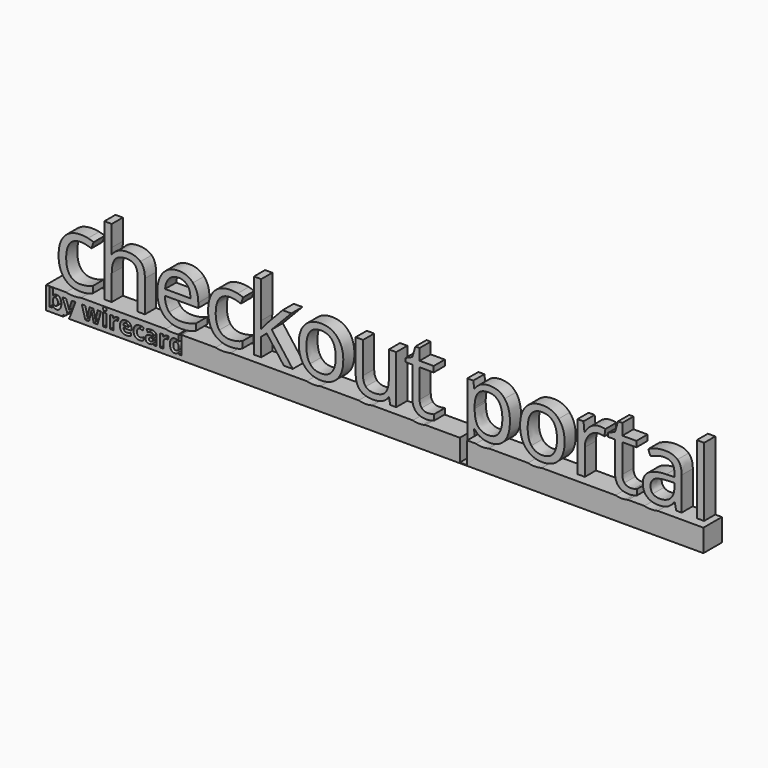
from build123d import *

# Parameters (mm, degrees)
F0_W         = 1.5870878906
F0_H         = 14.8709217956
F1_DEPTH     = 3
F2_DEPTH     = 5
F3_TEXT_SIZE = 4.9959736417
F4_DEPTH     = 2


# Not quite as in the source:
# - Text() gives the source's letters only with a copy of the font that has no kerning and outlines rounded to 1/6400 em; it was checked with that copy


with BuildPart() as f1:
    # F0 (on Front) → F1 (new body)
    with BuildSketch(Plane.XZ):
        with BuildLine():
            Line((-60.4767255251, 14.8709217956), (-60.4767255251, 0))
            Line((-60.4767255251, 0), (-58.8896376345, 0))
            Line((-58.8896376345, 0), (-58.8896376345, 5.4768293103))
            add(Edge.make_bspline(
                [(-58.1297313902, 8.4185991576), (-58.8896376345, 7.5195551502), (-58.8896376345, 5.4768293103)],
                knots=[0, 0, 0, 1, 1, 1], degree=2))
            add(Edge.make_bspline(
                [(-55.7185198261, 9.317643165), (-57.3698251458, 9.317643165), (-58.1297313902, 8.4185991576)],
                knots=[0, 0, 0, 1, 1, 1], degree=2))
            add(Edge.make_bspline(
                [(-53.8913810696, 8.6861717788), (-54.4739248908, 9.317643165), (-55.7185198261, 9.317643165)],
                knots=[0, 0, 0, 1, 1, 1], degree=2))
            add(Edge.make_bspline(
                [(-53.3088372485, 6.7764677563), (-53.3088372485, 8.0547003927), (-53.8913810696, 8.6861717788)],
                knots=[0, 0, 0, 1, 1, 1], degree=2))
            Line((-53.3088372485, 6.7764677563), (-53.3088372485, 0))
            Line((-53.3088372485, 0), (-51.721749358, 0))
            Line((-51.721749358, 0), (-51.721749358, 6.831511267))
            add(Edge.make_bspline(
                [(-52.683481808, 9.7319984813), (-51.721749358, 8.8191935962), (-51.721749358, 6.831511267)],
                knots=[0, 0, 0, 1, 1, 1], degree=2))
            add(Edge.make_bspline(
                [(-55.5656211854, 10.6448033663), (-53.6452142581, 10.6448033663), (-52.683481808, 9.7319984813)],
                knots=[0, 0, 0, 1, 1, 1], degree=2))
            add(Edge.make_bspline(
                [(-57.5380136506, 10.2105712267), (-56.6726073442, 10.6448033663), (-55.5656211854, 10.6448033663)],
                knots=[0, 0, 0, 1, 1, 1], degree=2))
            add(Edge.make_bspline(
                [(-58.8712897976, 9.021019802), (-58.403419957, 9.7763390871), (-57.5380136506, 10.2105712267)],
                knots=[0, 0, 0, 1, 1, 1], degree=2))
            Line((-58.8712897976, 9.021019802), (-58.9660869549, 9.021019802))
            add(Edge.make_bspline(
                [(-58.8896376345, 10.3695858131), (-58.8896376345, 9.5561650445), (-58.9660869549, 9.021019802)],
                knots=[0, 0, 0, 1, 1, 1], degree=2))
            Line((-58.8896376345, 10.3695858131), (-58.8896376345, 14.8709217956))
            Line((-58.8896376345, 14.8709217956), (-60.4767255251, 14.8709217956))
        make_face()
        with BuildLine():
            Line((-58.8896376345, 0), (-60.4767255251, 0))
            Line((-60.4767255251, 0), (-63.9066653381, 0))
            add(Edge.make_bspline(
                [(-63.9066653381, 0), (-64.6610084791, -0.1926522873), (-65.6080039074, -0.1926522873)],
                knots=[0.406741787, 0.406741787, 0.406741787, 1, 1, 1], degree=2))
            add(Edge.make_bspline(
                [(-65.6080039074, -0.1926522873), (-66.4518127873, -0.1926522873), (-67.1542872382, 0)],
                knots=[0, 0, 0, 0.3708835197, 0.3708835197, 0.3708835197], degree=2))
            Line((-67.1542872382, 0), (-71.4762537379, 0))
            Line((-71.4762537379, 0), (-71.4762537379, -4.8487260938))
            Line((-71.4762537379, -4.8487260938), (70.5573260784, -4.8487260938))
            Line((70.5573260784, -4.8487260938), (70.5573260784, 0))
            Line((70.5573260784, 0), (69.1171043692, 0))
            Line((69.1171043692, 0), (67.5300164786, 0))
            Line((67.5300164786, 0), (64.264101513, 0))
            Line((64.264101513, 0), (63.0867819795, 0))
            Line((63.0867819795, 0), (60.7063249973, 0))
            add(Edge.make_bspline(
                [(60.7063249973, 0), (60.0543585557, -0.1926522873), (59.1878666414, -0.1926522873)],
                knots=[0.2582329607, 0.2582329607, 0.2582329607, 1, 1, 1], degree=2))
            add(Edge.make_bspline(
                [(59.1878666414, -0.1926522873), (58.4260616691, -0.1926522873), (57.8254107013, 0)],
                knots=[0, 0, 0, 0.4894320446, 0.4894320446, 0.4894320446], degree=2))
            Line((57.8254107013, 0), (54.2992999583, 0))
            add(Edge.make_bspline(
                [(54.2992999583, 0), (54.0897603947, -0.0618327819), (53.7966605699, -0.1100870213)],
                knots=[0.4155624782, 0.4155624782, 0.4155624782, 1, 1, 1], degree=2))
            add(Edge.make_bspline(
                [(53.7966605699, -0.1100870213), (53.2951530284, -0.1926522873), (52.8915006169, -0.1926522873)],
                knots=[0, 0, 0, 1, 1, 1], degree=2))
            add(Edge.make_bspline(
                [(52.8915006169, -0.1926522873), (52.1466317843, -0.1926522873), (51.5844790179, 0)],
                knots=[0, 0, 0, 0.245299653, 0.245299653, 0.245299653], degree=2))
            Line((51.5844790179, 0), (43.3353355724, 0))
            Line((43.3353355724, 0), (41.7482476818, 0))
            Line((41.7482476818, 0), (35.6454867595, 0))
            add(Edge.make_bspline(
                [(35.6454867595, 0), (34.9450140523, -0.1926522873), (34.1124895647, -0.1926522873)],
                knots=[0.6340763655, 0.6340763655, 0.6340763655, 1, 1, 1], degree=2))
            add(Edge.make_bspline(
                [(34.1124895647, -0.1926522873), (33.3528022913, -0.1926522873), (32.6858735265, 0)],
                knots=[0, 0, 0, 0.5400617249, 0.5400617249, 0.5400617249], degree=2))
            Line((32.6858735265, 0), (24.1886250812, 0))
            add(Edge.make_bspline(
                [(24.1886250812, 0), (23.5581628048, -0.1926522873), (22.8071640705, -0.1926522873)],
                knots=[0.6329041565, 0.6329041565, 0.6329041565, 1, 1, 1], degree=2))
            add(Edge.make_bspline(
                [(22.8071640705, -0.1926522873), (22.0754941131, -0.1926522873), (21.4350805023, 0)],
                knots=[0, 0, 0, 0.714227875, 0.714227875, 0.714227875], degree=2))
            Line((21.4350805023, 0), (19.5134400115, 0))
            add(Edge.make_bspline(
                [(19.5134400115, 0), (19.5198432952, -0.1983221258), (19.5198432952, -0.3914205202)],
                knots=[0.7652569395, 0.7652569395, 0.7652569395, 1, 1, 1], degree=2))
            Line((19.5198432952, -0.3914205202), (19.5198432952, -4.7031621883))
            Line((19.5198432952, -4.7031621883), (17.9327554046, -4.7031621883))
            Line((17.9327554046, -4.7031621883), (17.9327554046, 0))
            Line((17.9327554046, 0), (10.4999553401, 0))
            add(Edge.make_bspline(
                [(10.4999553401, 0), (10.2904157764, -0.0618327819), (9.9973159517, -0.1100870213)],
                knots=[0.4155624782, 0.4155624782, 0.4155624782, 1, 1, 1], degree=2))
            add(Edge.make_bspline(
                [(9.9973159517, -0.1100870213), (9.4958084101, -0.1926522873), (9.0921559987, -0.1926522873)],
                knots=[0, 0, 0, 1, 1, 1], degree=2))
            add(Edge.make_bspline(
                [(9.0921559987, -0.1926522873), (8.3472871661, -0.1926522873), (7.7851343997, 0)],
                knots=[0, 0, 0, 0.245299653, 0.245299653, 0.245299653], degree=2))
            Line((7.7851343997, 0), (2.5756159315, 0))
            Line((2.5756159315, 0), (1.266803567, 0))
            Line((1.266803567, 0), (-0.9704054064, 0))
            add(Edge.make_bspline(
                [(-0.9704054064, 0), (-1.61552937, -0.1926522873), (-2.3752420547, -0.1926522873)],
                knots=[0.3156013684, 0.3156013684, 0.3156013684, 1, 1, 1], degree=2))
            add(Edge.make_bspline(
                [(-2.3752420547, -0.1926522873), (-3.2554913531, -0.1926522873), (-3.9317367984, 0)],
                knots=[0, 0, 0, 0.4605661865, 0.4605661865, 0.4605661865], degree=2))
            Line((-3.9317367984, 0), (-12.1750921094, 0))
            add(Edge.make_bspline(
                [(-12.1750921094, 0), (-12.8755648167, -0.1926522873), (-13.7080893043, -0.1926522873)],
                knots=[0.6340763655, 0.6340763655, 0.6340763655, 1, 1, 1], degree=2))
            add(Edge.make_bspline(
                [(-13.7080893043, -0.1926522873), (-14.4677765777, -0.1926522873), (-15.1347053424, 0)],
                knots=[0, 0, 0, 0.5400617249, 0.5400617249, 0.5400617249], degree=2))
            Line((-15.1347053424, 0), (-19.7842812861, 0))
            Line((-19.7842812861, 0), (-21.7046882135, 0))
            Line((-21.7046882135, 0), (-26.5974447162, 0))
            Line((-26.5974447162, 0), (-28.1661847699, 0))
            Line((-28.1661847699, 0), (-31.596124583, 0))
            add(Edge.make_bspline(
                [(-31.596124583, 0), (-32.3504677239, -0.1926522873), (-33.2974631522, -0.1926522873)],
                knots=[0.406741787, 0.406741787, 0.406741787, 1, 1, 1], degree=2))
            add(Edge.make_bspline(
                [(-33.2974631522, -0.1926522873), (-34.1412720322, -0.1926522873), (-34.843746483, 0)],
                knots=[0, 0, 0, 0.3708835197, 0.3708835197, 0.3708835197], degree=2))
            Line((-34.843746483, 0), (-42.0798203783, 0))
            add(Edge.make_bspline(
                [(-42.0798203783, 0), (-42.1552650705, -0.0178176726), (-42.2298017426, -0.033637701)],
                knots=[0.9005120931, 0.9005120931, 0.9005120931, 1, 1, 1], degree=2))
            add(Edge.make_bspline(
                [(-42.2298017426, -0.033637701), (-42.9790050821, -0.1926522873), (-44.0401216486, -0.1926522873)],
                knots=[0, 0, 0, 1, 1, 1], degree=2))
            add(Edge.make_bspline(
                [(-44.0401216486, -0.1926522873), (-44.896282125, -0.1926522873), (-45.6195000402, 0)],
                knots=[0, 0, 0, 0.3688754729, 0.3688754729, 0.3688754729], degree=2))
            Line((-45.6195000402, 0), (-51.721749358, 0))
            Line((-51.721749358, 0), (-53.3088372485, 0))
            Line((-53.3088372485, 0), (-58.8896376345, 0))
        make_face()
        with BuildLine():
            add(Edge.make_bspline(
                [(-63.9066653381, 0), (-64.6610084791, -0.1926522873), (-65.6080039074, -0.1926522873)],
                knots=[0.406741787, 0.406741787, 0.406741787, 1, 1, 1], degree=2))
            Line((-63.9066653381, 0), (-67.1542872382, 0))
            add(Edge.make_bspline(
                [(-65.6080039074, -0.1926522873), (-66.4518127873, -0.1926522873), (-67.1542872382, 0)],
                knots=[0, 0, 0, 0.3708835197, 0.3708835197, 0.3708835197], degree=2))
        make_face()
        with BuildLine():
            Line((-67.1542872382, 0), (-63.9066653381, 0))
            add(Edge.make_bspline(
                [(-62.9628574231, 0.3547248465), (-63.3894826503, 0.1320836929), (-63.9066653381, 0)],
                knots=[0, 0, 0, 0.406741787, 0.406741787, 0.406741787], degree=2))
            Line((-62.9628574231, 0.3547248465), (-62.9628574231, 1.7583343682))
            add(Edge.make_bspline(
                [(-65.647757554, 1.1956673704), (-64.3389451895, 1.1956673704), (-62.9628574231, 1.7583343682)],
                knots=[0, 0, 0, 1, 1, 1], degree=2))
            add(Edge.make_bspline(
                [(-67.9549980423, 2.2277331952), (-67.1767439611, 1.1956673704), (-65.647757554, 1.1956673704)],
                knots=[0, 0, 0, 1, 1, 1], degree=2))
            add(Edge.make_bspline(
                [(-68.7332521235, 5.1893798657), (-68.7332521235, 3.25979902), (-67.9549980423, 2.2277331952)],
                knots=[0, 0, 0, 1, 1, 1], degree=2))
            add(Edge.make_bspline(
                [(-65.5407285055, 9.2595416815), (-68.7332521235, 9.2595416815), (-68.7332521235, 5.1893798657)],
                knots=[0, 0, 0, 1, 1, 1], degree=2))
            add(Edge.make_bspline(
                [(-64.4429162651, 9.1219329048), (-65.0636847464, 9.2595416815), (-65.5407285055, 9.2595416815)],
                knots=[0, 0, 0, 1, 1, 1], degree=2))
            add(Edge.make_bspline(
                [(-63.2961764598, 8.773324004), (-63.8221477839, 8.9843241282), (-64.4429162651, 9.1219329048)],
                knots=[0, 0, 0, 1, 1, 1], degree=2))
            Line((-63.2961764598, 8.773324004), (-62.8099587824, 10.1188320423))
            add(Edge.make_bspline(
                [(-63.9933942615, 10.5026076305), (-63.2380749763, 10.3390060849), (-62.8099587824, 10.1188320423)],
                knots=[0, 0, 0, 1, 1, 1], degree=2))
            add(Edge.make_bspline(
                [(-65.5040328317, 10.666209176), (-64.7487135466, 10.666209176), (-63.9933942615, 10.5026076305)],
                knots=[0, 0, 0, 1, 1, 1], degree=2))
            add(Edge.make_bspline(
                [(-69.1109117661, 9.2320199262), (-67.8433820346, 10.666209176), (-65.5040328317, 10.666209176)],
                knots=[0, 0, 0, 1, 1, 1], degree=2))
            add(Edge.make_bspline(
                [(-70.3784414976, 5.1710320289), (-70.3784414976, 7.7978306763), (-69.1109117661, 9.2320199262)],
                knots=[0, 0, 0, 1, 1, 1], degree=2))
            add(Edge.make_bspline(
                [(-69.1307885894, 1.2078992616), (-70.3784414976, 2.6084508105), (-70.3784414976, 5.1710320289)],
                knots=[0, 0, 0, 1, 1, 1], degree=2))
            add(Edge.make_bspline(
                [(-67.1542872382, 0), (-68.3458695831, 0.3267892006), (-69.1307885894, 1.2078992616)],
                knots=[0.3708835197, 0.3708835197, 0.3708835197, 1, 1, 1], degree=2))
        make_face()
        with BuildLine():
            add(Edge.make_bspline(
                [(-45.6195000402, 0), (-46.8568839229, 0.3296168834), (-47.7051020665, 1.2231891257)],
                knots=[0.3688754729, 0.3688754729, 0.3688754729, 1, 1, 1], degree=2))
            Line((-45.6195000402, 0), (-42.0798203783, 0))
            add(Edge.make_bspline(
                [(-40.6396558792, 0.4862176775), (-41.3969347915, 0.1612761805), (-42.0798203783, 0)],
                knots=[0, 0, 0, 0.9005120931, 0.9005120931, 0.9005120931], degree=2))
            Line((-40.6396558792, 0.4862176775), (-40.6396558792, 1.9020590905))
            add(Edge.make_bspline(
                [(-43.9820201651, 1.1956673704), (-42.2909611989, 1.1956673704), (-40.6396558792, 1.9020590905)],
                knots=[0, 0, 0, 1, 1, 1], degree=2))
            add(Edge.make_bspline(
                [(-46.4712100359, 2.1512838748), (-45.5874558926, 1.1956673704), (-43.9820201651, 1.1956673704)],
                knots=[0, 0, 0, 1, 1, 1], degree=2))
            add(Edge.make_bspline(
                [(-47.4038917443, 4.9508579862), (-47.3549641792, 3.1069003793), (-46.4712100359, 2.1512838748)],
                knots=[0, 0, 0, 1, 1, 1], degree=2))
            Line((-47.4038917443, 4.9508579862), (-40.1901338755, 4.9508579862))
            Line((-40.1901338755, 4.9508579862), (-40.1901338755, 5.9538730693))
            add(Edge.make_bspline(
                [(-41.3368736808, 9.3711576892), (-40.1901338755, 8.0761062024), (-40.1901338755, 5.9538730693)],
                knots=[0, 0, 0, 1, 1, 1], degree=2))
            add(Edge.make_bspline(
                [(-44.4498900057, 10.666209176), (-42.4836134862, 10.666209176), (-41.3368736808, 9.3711576892)],
                knots=[0, 0, 0, 1, 1, 1], degree=2))
            add(Edge.make_bspline(
                [(-47.8014282101, 9.1754474291), (-46.5537753019, 10.666209176), (-44.4498900057, 10.666209176)],
                knots=[0, 0, 0, 1, 1, 1], degree=2))
            add(Edge.make_bspline(
                [(-49.0490811183, 5.1496262192), (-49.0490811183, 7.6846856822), (-47.8014282101, 9.1754474291)],
                knots=[0, 0, 0, 1, 1, 1], degree=2))
            add(Edge.make_bspline(
                [(-47.7051020665, 1.2231891257), (-49.0490811183, 2.6390305387), (-49.0490811183, 5.1496262192)],
                knots=[0, 0, 0, 1, 1, 1], degree=2))
        make_face()
        with BuildLine():
            add(Edge.make_bspline(
                [(-44.4712958154, 9.3359910018), (-45.7311806149, 9.3359910018), (-46.4819129408, 8.5149253012)],
                knots=[0, 0, 0, 1, 1, 1], degree=2))
            add(Edge.make_bspline(
                [(-42.5585338201, 8.5378600973), (-43.22670088, 9.3359910018), (-44.4712958154, 9.3359910018)],
                knots=[0, 0, 0, 1, 1, 1], degree=2))
            add(Edge.make_bspline(
                [(-41.8903667602, 6.2413225138), (-41.8903667602, 7.7397291928), (-42.5585338201, 8.5378600973)],
                knots=[0, 0, 0, 1, 1, 1], degree=2))
            Line((-41.8903667602, 6.2413225138), (-47.3671960705, 6.2413225138))
            add(Edge.make_bspline(
                [(-46.4819129408, 8.5149253012), (-47.2326452667, 7.6938596006), (-47.3671960705, 6.2413225138)],
                knots=[0, 0, 0, 1, 1, 1], degree=2))
        make_face(mode=Mode.SUBTRACT)
        with BuildLine():
            Line((-42.0798203783, 0), (-45.6195000402, 0))
            add(Edge.make_bspline(
                [(-44.0401216486, -0.1926522873), (-44.896282125, -0.1926522873), (-45.6195000402, 0)],
                knots=[0, 0, 0, 0.3688754729, 0.3688754729, 0.3688754729], degree=2))
            add(Edge.make_bspline(
                [(-42.2298017426, -0.033637701), (-42.9790050821, -0.1926522873), (-44.0401216486, -0.1926522873)],
                knots=[0, 0, 0, 1, 1, 1], degree=2))
            add(Edge.make_bspline(
                [(-42.0798203783, 0), (-42.1552650705, -0.0178176726), (-42.2298017426, -0.033637701)],
                knots=[0.9005120931, 0.9005120931, 0.9005120931, 1, 1, 1], degree=2))
        make_face()
        with BuildLine():
            add(Edge.make_bspline(
                [(-34.843746483, 0), (-36.0353288279, 0.3267892006), (-36.8202478342, 1.2078992616)],
                knots=[0.3708835197, 0.3708835197, 0.3708835197, 1, 1, 1], degree=2))
            Line((-34.843746483, 0), (-31.596124583, 0))
            add(Edge.make_bspline(
                [(-30.6523166679, 0.3547248465), (-31.0789418951, 0.1320836929), (-31.596124583, 0)],
                knots=[0, 0, 0, 0.406741787, 0.406741787, 0.406741787], degree=2))
            Line((-30.6523166679, 0.3547248465), (-30.6523166679, 1.7583343682))
            add(Edge.make_bspline(
                [(-33.3372167988, 1.1956673704), (-32.0284044343, 1.1956673704), (-30.6523166679, 1.7583343682)],
                knots=[0, 0, 0, 1, 1, 1], degree=2))
            add(Edge.make_bspline(
                [(-35.6444572871, 2.2277331952), (-34.8662032059, 1.1956673704), (-33.3372167988, 1.1956673704)],
                knots=[0, 0, 0, 1, 1, 1], degree=2))
            add(Edge.make_bspline(
                [(-36.4227113684, 5.1893798657), (-36.4227113684, 3.25979902), (-35.6444572871, 2.2277331952)],
                knots=[0, 0, 0, 1, 1, 1], degree=2))
            add(Edge.make_bspline(
                [(-33.2301877503, 9.2595416815), (-36.4227113684, 9.2595416815), (-36.4227113684, 5.1893798657)],
                knots=[0, 0, 0, 1, 1, 1], degree=2))
            add(Edge.make_bspline(
                [(-32.13237551, 9.1219329048), (-32.7531439913, 9.2595416815), (-33.2301877503, 9.2595416815)],
                knots=[0, 0, 0, 1, 1, 1], degree=2))
            add(Edge.make_bspline(
                [(-30.9856357047, 8.773324004), (-31.5116070287, 8.9843241282), (-32.13237551, 9.1219329048)],
                knots=[0, 0, 0, 1, 1, 1], degree=2))
            Line((-30.9856357047, 8.773324004), (-30.4994180272, 10.1188320423))
            add(Edge.make_bspline(
                [(-31.6828535063, 10.5026076305), (-30.9275342212, 10.3390060849), (-30.4994180272, 10.1188320423)],
                knots=[0, 0, 0, 1, 1, 1], degree=2))
            add(Edge.make_bspline(
                [(-33.1934920765, 10.666209176), (-32.4381727914, 10.666209176), (-31.6828535063, 10.5026076305)],
                knots=[0, 0, 0, 1, 1, 1], degree=2))
            add(Edge.make_bspline(
                [(-36.8003710109, 9.2320199262), (-35.5328412794, 10.666209176), (-33.1934920765, 10.666209176)],
                knots=[0, 0, 0, 1, 1, 1], degree=2))
            add(Edge.make_bspline(
                [(-38.0679007424, 5.1710320289), (-38.0679007424, 7.7978306763), (-36.8003710109, 9.2320199262)],
                knots=[0, 0, 0, 1, 1, 1], degree=2))
            add(Edge.make_bspline(
                [(-36.8202478342, 1.2078992616), (-38.0679007424, 2.6084508105), (-38.0679007424, 5.1710320289)],
                knots=[0, 0, 0, 1, 1, 1], degree=2))
        make_face()
        with BuildLine():
            Line((-31.596124583, 0), (-34.843746483, 0))
            add(Edge.make_bspline(
                [(-33.2974631522, -0.1926522873), (-34.1412720322, -0.1926522873), (-34.843746483, 0)],
                knots=[0, 0, 0, 0.3708835197, 0.3708835197, 0.3708835197], degree=2))
            add(Edge.make_bspline(
                [(-31.596124583, 0), (-32.3504677239, -0.1926522873), (-33.2974631522, -0.1926522873)],
                knots=[0.406741787, 0.406741787, 0.406741787, 1, 1, 1], degree=2))
        make_face()
        with Locations((68.3235604239, 7.4354608978)):
            Rectangle(F0_W, F0_H)
        with BuildLine():
            Line((-28.1661847699, 14.8709217956), (-28.1661847699, 0))
            Line((-28.1661847699, 0), (-26.5974447162, 0))
            Line((-26.5974447162, 0), (-26.5974447162, 3.917263175))
            Line((-26.5974447162, 3.917263175), (-25.4048353187, 4.9508579862))
            Line((-25.4048353187, 4.9508579862), (-21.7046882135, 0))
            Line((-21.7046882135, 0), (-19.7842812861, 0))
            Line((-19.7842812861, 0), (-24.3253709153, 6.0119745528))
            Line((-24.3253709153, 6.0119745528), (-20.0809046491, 10.4735568887))
            Line((-20.0809046491, 10.4735568887), (-21.9646159027, 10.4735568887))
            Line((-21.9646159027, 10.4735568887), (-25.3467338352, 6.8896127505))
            add(Edge.make_bspline(
                [(-26.5974447162, 5.3606263433), (-26.1876763591, 5.9446991509), (-25.3467338352, 6.8896127505)],
                knots=[0, 0, 0, 1, 1, 1], degree=2))
            Line((-26.5974447162, 5.3606263433), (-26.6738940366, 5.3606263433))
            add(Edge.make_bspline(
                [(-26.5974447162, 6.9844099077), (-26.5974447162, 6.4614965565), (-26.6738940366, 5.3606263433)],
                knots=[0, 0, 0, 1, 1, 1], degree=2))
            Line((-26.5974447162, 6.9844099077), (-26.5974447162, 14.8709217956))
            Line((-26.5974447162, 14.8709217956), (-28.1661847699, 14.8709217956))
        make_face()
        with BuildLine():
            Line((63.0867819795, 0), (64.264101513, 0))
            Line((64.264101513, 0), (64.264101513, 7.1495404397))
            add(Edge.make_bspline(
                [(63.3604705464, 9.8145637473), (64.264101513, 8.9843241282), (64.264101513, 7.1495404397)],
                knots=[0, 0, 0, 1, 1, 1], degree=2))
            add(Edge.make_bspline(
                [(60.5853602175, 10.6448033663), (62.4568395798, 10.6448033663), (63.3604705464, 9.8145637473)],
                knots=[0, 0, 0, 1, 1, 1], degree=2))
            add(Edge.make_bspline(
                [(58.7337576785, 10.4062814868), (59.655736482, 10.6448033663), (60.5853602175, 10.6448033663)],
                knots=[0, 0, 0, 1, 1, 1], degree=2))
            add(Edge.make_bspline(
                [(57.038111753, 9.7488173318), (57.811778875, 10.1677596073), (58.7337576785, 10.4062814868)],
                knots=[0, 0, 0, 1, 1, 1], degree=2))
            Line((57.038111753, 9.7488173318), (57.5273874032, 8.5348021245))
            add(Edge.make_bspline(
                [(60.4875050874, 9.3359910018), (59.1786927229, 9.3359910018), (57.5273874032, 8.5348021245)],
                knots=[0, 0, 0, 1, 1, 1], degree=2))
            add(Edge.make_bspline(
                [(62.1846799993, 8.7488602215), (61.6556507025, 9.3359910018), (60.4875050874, 9.3359910018)],
                knots=[0, 0, 0, 1, 1, 1], degree=2))
            add(Edge.make_bspline(
                [(62.7137092962, 6.929366397), (62.7137092962, 8.1617294412), (62.1846799993, 8.7488602215)],
                knots=[0, 0, 0, 1, 1, 1], degree=2))
            Line((62.7137092962, 6.929366397), (62.7137092962, 6.2780181876))
            Line((62.7137092962, 6.2780181876), (60.9370270911, 6.2199167041))
            add(Edge.make_bspline(
                [(55.8638501923, 2.8959002551), (55.8638501923, 6.0670180634), (60.9370270911, 6.2199167041)],
                knots=[0, 0, 0, 1, 1, 1], degree=2))
            add(Edge.make_bspline(
                [(56.7476043356, 0.6115945628), (55.8638501923, 1.415841413), (55.8638501923, 2.8959002551)],
                knots=[0, 0, 0, 1, 1, 1], degree=2))
            add(Edge.make_bspline(
                [(57.8254107013, 0), (57.1988208817, 0.2009718929), (56.7476043356, 0.6115945628)],
                knots=[0.4894320446, 0.4894320446, 0.4894320446, 1, 1, 1], degree=2))
            Line((57.8254107013, 0), (60.7063249973, 0))
            add(Edge.make_bspline(
                [(61.1342663376, 0.1574855999), (60.9332954821, 0.0670684567), (60.7063249973, 0)],
                knots=[0, 0, 0, 0.2582329607, 0.2582329607, 0.2582329607], degree=2))
            add(Edge.make_bspline(
                [(62.6953614593, 1.4922907333), (61.9125204189, 0.5076234872), (61.1342663376, 0.1574855999)],
                knots=[0, 0, 0, 1, 1, 1], degree=2))
            Line((62.6953614593, 1.4922907333), (62.7718107797, 1.4922907333))
            Line((62.7718107797, 1.4922907333), (63.0867819795, 0))
        make_face()
        with BuildLine():
            add(Edge.make_bspline(
                [(59.5028378412, 1.11921805), (60.9859546561, 1.11921805), (61.8314841393, 1.9311098322)],
                knots=[0, 0, 0, 1, 1, 1], degree=2))
            add(Edge.make_bspline(
                [(58.0472427817, 1.5672110673), (58.5670981601, 1.11921805), (59.5028378412, 1.11921805)],
                knots=[0, 0, 0, 1, 1, 1], degree=2))
            add(Edge.make_bspline(
                [(57.5273874032, 2.8775524182), (57.5273874032, 2.0152040846), (58.0472427817, 1.5672110673)],
                knots=[0, 0, 0, 1, 1, 1], degree=2))
            add(Edge.make_bspline(
                [(58.3622139815, 4.4967490233), (57.5273874032, 3.9753646585), (57.5273874032, 2.8775524182)],
                knots=[0, 0, 0, 1, 1, 1], degree=2))
            add(Edge.make_bspline(
                [(61.0899257318, 5.0854087901), (59.1970405598, 5.0181333882), (58.3622139815, 4.4967490233)],
                knots=[0, 0, 0, 1, 1, 1], degree=2))
            Line((61.0899257318, 5.0854087901), (62.6770136224, 5.1496262192))
            Line((62.6770136224, 5.1496262192), (62.6770136224, 4.2047126196))
            add(Edge.make_bspline(
                [(61.8314841393, 1.9311098322), (62.6770136224, 2.7430016144), (62.6770136224, 4.2047126196)],
                knots=[0, 0, 0, 1, 1, 1], degree=2))
        make_face(mode=Mode.SUBTRACT)
        with BuildLine():
            add(Edge.make_bspline(
                [(60.7063249973, 0), (60.0543585557, -0.1926522873), (59.1878666414, -0.1926522873)],
                knots=[0.2582329607, 0.2582329607, 0.2582329607, 1, 1, 1], degree=2))
            Line((60.7063249973, 0), (57.8254107013, 0))
            add(Edge.make_bspline(
                [(59.1878666414, -0.1926522873), (58.4260616691, -0.1926522873), (57.8254107013, 0)],
                knots=[0, 0, 0, 0.4894320446, 0.4894320446, 0.4894320446], degree=2))
        make_face()
        with BuildLine():
            add(Edge.make_bspline(
                [(-15.1347053424, 0), (-15.7026886887, 0.1640704324), (-16.2033951207, 0.4678698406)],
                knots=[0.5400617249, 0.5400617249, 0.5400617249, 1, 1, 1], degree=2))
            Line((-15.1347053424, 0), (-12.1750921094, 0))
            add(Edge.make_bspline(
                [(-10.1440219893, 1.2461239218), (-10.9613055526, 0.3338299323), (-12.1750921094, 0)],
                knots=[0, 0, 0, 0.6340763655, 0.6340763655, 0.6340763655], degree=2))
            add(Edge.make_bspline(
                [(-8.8550864481, 5.2474813492), (-8.8550864481, 2.6849001309), (-10.1440219893, 1.2461239218)],
                knots=[0, 0, 0, 1, 1, 1], degree=2))
            add(Edge.make_bspline(
                [(-10.1501379349, 9.2029691844), (-8.8550864481, 7.7397291928), (-8.8550864481, 5.2474813492)],
                knots=[0, 0, 0, 1, 1, 1], degree=2))
            add(Edge.make_bspline(
                [(-13.6408139023, 10.666209176), (-11.4451894217, 10.666209176), (-10.1501379349, 9.2029691844)],
                knots=[0, 0, 0, 1, 1, 1], degree=2))
            add(Edge.make_bspline(
                [(-17.1972362853, 9.2366068854), (-15.9159456761, 10.666209176), (-13.6408139023, 10.666209176)],
                knots=[0, 0, 0, 1, 1, 1], degree=2))
            add(Edge.make_bspline(
                [(-18.4785268944, 5.2474813492), (-18.4785268944, 7.8070045947), (-17.1972362853, 9.2366068854)],
                knots=[0, 0, 0, 1, 1, 1], degree=2))
            add(Edge.make_bspline(
                [(-17.8852801685, 2.3607550126), (-18.4785268944, 3.5931180567), (-18.4785268944, 5.2474813492)],
                knots=[0, 0, 0, 1, 1, 1], degree=2))
            add(Edge.make_bspline(
                [(-16.2033951207, 0.4678698406), (-17.2920334425, 1.1283919685), (-17.8852801685, 2.3607550126)],
                knots=[0, 0, 0, 1, 1, 1], degree=2))
        make_face()
        with BuildLine():
            add(Edge.make_bspline(
                [(-16.8333375204, 5.2474813492), (-16.8333375204, 3.2383932103), (-16.0306196567, 2.1879795486)],
                knots=[0, 0, 0, 1, 1, 1], degree=2))
            add(Edge.make_bspline(
                [(-16.0397935751, 8.2947512586), (-16.8333375204, 7.2718593522), (-16.8333375204, 5.2474813492)],
                knots=[0, 0, 0, 1, 1, 1], degree=2))
            add(Edge.make_bspline(
                [(-13.6897414674, 9.317643165), (-15.2462496298, 9.317643165), (-16.0397935751, 8.2947512586)],
                knots=[0, 0, 0, 1, 1, 1], degree=2))
            add(Edge.make_bspline(
                [(-11.3045226723, 8.2809903809), (-12.1118274952, 9.317643165), (-13.6897414674, 9.317643165)],
                knots=[0, 0, 0, 1, 1, 1], degree=2))
            add(Edge.make_bspline(
                [(-10.4972178493, 5.2474813492), (-10.4972178493, 7.2443375969), (-11.3045226723, 8.2809903809)],
                knots=[0, 0, 0, 1, 1, 1], degree=2))
            add(Edge.make_bspline(
                [(-11.3045226723, 2.1833925894), (-10.4972178493, 3.2292192918), (-10.4972178493, 5.2474813492)],
                knots=[0, 0, 0, 1, 1, 1], degree=2))
            add(Edge.make_bspline(
                [(-13.6713936305, 1.1375658869), (-12.1118274952, 1.1375658869), (-11.3045226723, 2.1833925894)],
                knots=[0, 0, 0, 1, 1, 1], degree=2))
            add(Edge.make_bspline(
                [(-16.0306196567, 2.1879795486), (-15.2279017929, 1.1375658869), (-13.6713936305, 1.1375658869)],
                knots=[0, 0, 0, 1, 1, 1], degree=2))
        make_face(mode=Mode.SUBTRACT)
        with BuildLine():
            Line((-12.1750921094, 0), (-15.1347053424, 0))
            add(Edge.make_bspline(
                [(-13.7080893043, -0.1926522873), (-14.4677765777, -0.1926522873), (-15.1347053424, 0)],
                knots=[0, 0, 0, 0.5400617249, 0.5400617249, 0.5400617249], degree=2))
            add(Edge.make_bspline(
                [(-12.1750921094, 0), (-12.8755648167, -0.1926522873), (-13.7080893043, -0.1926522873)],
                knots=[0.6340763655, 0.6340763655, 0.6340763655, 1, 1, 1], degree=2))
        make_face()
        with BuildLine():
            add(Edge.make_bspline(
                [(54.2992999583, 0), (54.0897603947, -0.0618327819), (53.7966605699, -0.1100870213)],
                knots=[0.4155624782, 0.4155624782, 0.4155624782, 1, 1, 1], degree=2))
            Line((54.2992999583, 0), (51.5844790179, 0))
            add(Edge.make_bspline(
                [(52.8915006169, -0.1926522873), (52.1466317843, -0.1926522873), (51.5844790179, 0)],
                knots=[0, 0, 0, 0.245299653, 0.245299653, 0.245299653], degree=2))
            add(Edge.make_bspline(
                [(53.7966605699, -0.1100870213), (53.2951530284, -0.1926522873), (52.8915006169, -0.1926522873)],
                knots=[0, 0, 0, 1, 1, 1], degree=2))
        make_face()
        with BuildLine():
            Line((51.5844790179, 0), (54.2992999583, 0))
            add(Edge.make_bspline(
                [(54.5550378278, 0.0947971572), (54.4482924119, 0.0439660068), (54.2992999583, 0)],
                knots=[0, 0, 0, 0.4155624782, 0.4155624782, 0.4155624782], degree=2))
            Line((54.5550378278, 0.0947971572), (54.5550378278, 1.3088123645))
            add(Edge.make_bspline(
                [(53.9342693465, 1.1803775063), (54.3256898668, 1.2415369626), (54.5550378278, 1.3088123645)],
                knots=[0, 0, 0, 1, 1, 1], degree=2))
            add(Edge.make_bspline(
                [(53.1208485779, 1.11921805), (53.5428488263, 1.11921805), (53.9342693465, 1.1803775063)],
                knots=[0, 0, 0, 1, 1, 1], degree=2))
            add(Edge.make_bspline(
                [(51.8884855338, 1.6253125508), (52.3380075375, 1.11921805), (53.1208485779, 1.11921805)],
                knots=[0, 0, 0, 1, 1, 1], degree=2))
            add(Edge.make_bspline(
                [(51.4389635301, 3.0763206511), (51.4389635301, 2.1314070515), (51.8884855338, 1.6253125508)],
                knots=[0, 0, 0, 1, 1, 1], degree=2))
            Line((51.4389635301, 3.0763206511), (51.4389635301, 9.2411938446))
            Line((51.4389635301, 9.2411938446), (54.4785885075, 9.2411938446))
            Line((54.4785885075, 9.2411938446), (54.4785885075, 10.4735568887))
            Line((54.4785885075, 10.4735568887), (51.4389635301, 10.4735568887))
            Line((51.4389635301, 10.4735568887), (51.4389635301, 12.9015873032))
            Line((51.4389635301, 12.9015873032), (50.5215716858, 12.9015873032))
            Line((50.5215716858, 12.9015873032), (49.8549336123, 10.666209176))
            Line((49.8549336123, 10.666209176), (48.3534689606, 10.0056870482))
            Line((48.3534689606, 10.0056870482), (48.3534689606, 9.2411938446))
            Line((48.3534689606, 9.2411938446), (49.8549336123, 9.2411938446))
            Line((49.8549336123, 9.2411938446), (49.8549336123, 3.0090452492))
            add(Edge.make_bspline(
                [(51.5844790179, 0), (49.8549336123, 0.5927230075), (49.8549336123, 3.0090452492)],
                knots=[0.245299653, 0.245299653, 0.245299653, 1, 1, 1], degree=2))
        make_face()
        with BuildLine():
            add(Edge.make_bspline(
                [(-3.9317367984, 0), (-4.723782915, 0.2256421793), (-5.2359756224, 0.7155656385)],
                knots=[0.4605661865, 0.4605661865, 0.4605661865, 1, 1, 1], degree=2))
            Line((-3.9317367984, 0), (-0.9704054064, 0))
            add(Edge.make_bspline(
                [(-0.3997916167, 0.2186450562), (-0.6729150312, 0.0888390518), (-0.9704054064, 0)],
                knots=[0, 0, 0, 0.3156013684, 0.3156013684, 0.3156013684], degree=2))
            add(Edge.make_bspline(
                [(0.9518323672, 1.4036095217), (0.4656146897, 0.6299423997), (-0.3997916167, 0.2186450562)],
                knots=[0, 0, 0, 1, 1, 1], degree=2))
            Line((0.9518323672, 1.4036095217), (1.037455606, 1.4036095217))
            Line((1.037455606, 1.4036095217), (1.266803567, 0))
            Line((1.266803567, 0), (2.5756159315, 0))
            Line((2.5756159315, 0), (2.5756159315, 10.4735568887))
            Line((2.5756159315, 10.4735568887), (0.9885280409, 10.4735568887))
            Line((0.9885280409, 10.4735568887), (0.9885280409, 4.9692058231))
            add(Edge.make_bspline(
                [(0.230150783, 2.0350809079), (0.9885280409, 2.9325959288), (0.9885280409, 4.9692058231)],
                knots=[0, 0, 0, 1, 1, 1], degree=2))
            add(Edge.make_bspline(
                [(-2.173415849, 1.1375658869), (-0.5282264749, 1.1375658869), (0.230150783, 2.0350809079)],
                knots=[0, 0, 0, 1, 1, 1], degree=2))
            add(Edge.make_bspline(
                [(-3.9974966327, 1.7675082866), (-3.4149528116, 1.1375658869), (-2.173415849, 1.1375658869)],
                knots=[0, 0, 0, 1, 1, 1], degree=2))
            add(Edge.make_bspline(
                [(-4.5800404538, 3.6787412955), (-4.5800404538, 2.3974506864), (-3.9974966327, 1.7675082866)],
                knots=[0, 0, 0, 1, 1, 1], degree=2))
            Line((-4.5800404538, 3.6787412955), (-4.5800404538, 10.4735568887))
            Line((-4.5800404538, 10.4735568887), (-6.1854761812, 10.4735568887))
            Line((-6.1854761812, 10.4735568887), (-6.1854761812, 3.620639812))
            add(Edge.make_bspline(
                [(-5.2359756224, 0.7155656385), (-6.1854761812, 1.6237835644), (-6.1854761812, 3.620639812)],
                knots=[0, 0, 0, 1, 1, 1], degree=2))
        make_face()
        with BuildLine():
            Line((-0.9704054064, 0), (-3.9317367984, 0))
            add(Edge.make_bspline(
                [(-2.3752420547, -0.1926522873), (-3.2554913531, -0.1926522873), (-3.9317367984, 0)],
                knots=[0, 0, 0, 0.4605661865, 0.4605661865, 0.4605661865], degree=2))
            add(Edge.make_bspline(
                [(-0.9704054064, 0), (-1.61552937, -0.1926522873), (-2.3752420547, -0.1926522873)],
                knots=[0.3156013684, 0.3156013684, 0.3156013684, 1, 1, 1], degree=2))
        make_face()
        with BuildLine():
            Line((41.7482476818, 0), (43.3353355724, 0))
            Line((43.3353355724, 0), (43.3353355724, 5.6205540326))
            add(Edge.make_bspline(
                [(44.2374375526, 8.1907801829), (43.3353355724, 7.1587143581), (43.3353355724, 5.6205540326)],
                knots=[0, 0, 0, 1, 1, 1], degree=2))
            add(Edge.make_bspline(
                [(46.4116562235, 9.2228460077), (45.1395395328, 9.2228460077), (44.2374375526, 8.1907801829)],
                knots=[0, 0, 0, 1, 1, 1], degree=2))
            add(Edge.make_bspline(
                [(47.5583960289, 9.0791212855), (46.9101057922, 9.2228460077), (46.4116562235, 9.2228460077)],
                knots=[0, 0, 0, 1, 1, 1], degree=2))
            Line((47.5583960289, 9.0791212855), (47.7785700715, 10.5500062091))
            add(Edge.make_bspline(
                [(46.5278591905, 10.666209176), (47.2250769921, 10.666209176), (47.7785700715, 10.5500062091)],
                knots=[0, 0, 0, 1, 1, 1], degree=2))
            add(Edge.make_bspline(
                [(44.7205972573, 10.1111871103), (45.5431919443, 10.666209176), (46.5278591905, 10.666209176)],
                knots=[0, 0, 0, 1, 1, 1], degree=2))
            add(Edge.make_bspline(
                [(43.3169877355, 8.5348021245), (43.8980025702, 9.5561650445), (44.7205972573, 10.1111871103)],
                knots=[0, 0, 0, 1, 1, 1], degree=2))
            Line((43.3169877355, 8.5348021245), (43.2405384152, 8.5348021245))
            Line((43.2405384152, 8.5348021245), (43.0570600463, 10.4735568887))
            Line((43.0570600463, 10.4735568887), (41.7482476818, 10.4735568887))
            Line((41.7482476818, 10.4735568887), (41.7482476818, 0))
        make_face()
        with BuildLine():
            add(Edge.make_bspline(
                [(35.6454867595, 0), (34.9450140523, -0.1926522873), (34.1124895647, -0.1926522873)],
                knots=[0.6340763655, 0.6340763655, 0.6340763655, 1, 1, 1], degree=2))
            Line((35.6454867595, 0), (32.6858735265, 0))
            add(Edge.make_bspline(
                [(34.1124895647, -0.1926522873), (33.3528022913, -0.1926522873), (32.6858735265, 0)],
                knots=[0, 0, 0, 0.5400617249, 0.5400617249, 0.5400617249], degree=2))
        make_face()
        with BuildLine():
            Line((32.6858735265, 0), (35.6454867595, 0))
            add(Edge.make_bspline(
                [(37.6765568797, 1.2461239218), (36.8592733163, 0.3338299323), (35.6454867595, 0)],
                knots=[0, 0, 0, 0.6340763655, 0.6340763655, 0.6340763655], degree=2))
            add(Edge.make_bspline(
                [(38.9654924209, 5.2474813492), (38.9654924209, 2.6849001309), (37.6765568797, 1.2461239218)],
                knots=[0, 0, 0, 1, 1, 1], degree=2))
            add(Edge.make_bspline(
                [(37.670440934, 9.2029691844), (38.9654924209, 7.7397291928), (38.9654924209, 5.2474813492)],
                knots=[0, 0, 0, 1, 1, 1], degree=2))
            add(Edge.make_bspline(
                [(34.1797649666, 10.666209176), (36.3753894472, 10.666209176), (37.670440934, 9.2029691844)],
                knots=[0, 0, 0, 1, 1, 1], degree=2))
            add(Edge.make_bspline(
                [(30.6233425836, 9.2366068854), (31.9046331928, 10.666209176), (34.1797649666, 10.666209176)],
                knots=[0, 0, 0, 1, 1, 1], degree=2))
            add(Edge.make_bspline(
                [(29.3420519745, 5.2474813492), (29.3420519745, 7.8070045947), (30.6233425836, 9.2366068854)],
                knots=[0, 0, 0, 1, 1, 1], degree=2))
            add(Edge.make_bspline(
                [(29.9352987004, 2.3607550126), (29.3420519745, 3.5931180567), (29.3420519745, 5.2474813492)],
                knots=[0, 0, 0, 1, 1, 1], degree=2))
            add(Edge.make_bspline(
                [(31.6171837483, 0.4678698406), (30.5285454264, 1.1283919685), (29.9352987004, 2.3607550126)],
                knots=[0, 0, 0, 1, 1, 1], degree=2))
            add(Edge.make_bspline(
                [(32.6858735265, 0), (32.1178901803, 0.1640704324), (31.6171837483, 0.4678698406)],
                knots=[0.5400617249, 0.5400617249, 0.5400617249, 1, 1, 1], degree=2))
        make_face()
        with BuildLine():
            add(Edge.make_bspline(
                [(30.9872413485, 5.2474813492), (30.9872413485, 3.2383932103), (31.7899592123, 2.1879795486)],
                knots=[0, 0, 0, 1, 1, 1], degree=2))
            add(Edge.make_bspline(
                [(31.7807852938, 8.2947512586), (30.9872413485, 7.2718593522), (30.9872413485, 5.2474813492)],
                knots=[0, 0, 0, 1, 1, 1], degree=2))
            add(Edge.make_bspline(
                [(34.1308374016, 9.317643165), (32.5743292391, 9.317643165), (31.7807852938, 8.2947512586)],
                knots=[0, 0, 0, 1, 1, 1], degree=2))
            add(Edge.make_bspline(
                [(36.5160561967, 8.2809903809), (35.7087513737, 9.317643165), (34.1308374016, 9.317643165)],
                knots=[0, 0, 0, 1, 1, 1], degree=2))
            add(Edge.make_bspline(
                [(37.3233610196, 5.2474813492), (37.3233610196, 7.2443375969), (36.5160561967, 8.2809903809)],
                knots=[0, 0, 0, 1, 1, 1], degree=2))
            add(Edge.make_bspline(
                [(36.5160561967, 2.1833925894), (37.3233610196, 3.2292192918), (37.3233610196, 5.2474813492)],
                knots=[0, 0, 0, 1, 1, 1], degree=2))
            add(Edge.make_bspline(
                [(34.1491852385, 1.1375658869), (35.7087513737, 1.1375658869), (36.5160561967, 2.1833925894)],
                knots=[0, 0, 0, 1, 1, 1], degree=2))
            add(Edge.make_bspline(
                [(31.7899592123, 2.1879795486), (32.592677076, 1.1375658869), (34.1491852385, 1.1375658869)],
                knots=[0, 0, 0, 1, 1, 1], degree=2))
        make_face(mode=Mode.SUBTRACT)
        with BuildLine():
            add(Edge.make_bspline(
                [(7.7851343997, 0), (6.0555889941, 0.5927230075), (6.0555889941, 3.0090452492)],
                knots=[0.245299653, 0.245299653, 0.245299653, 1, 1, 1], degree=2))
            Line((7.7851343997, 0), (10.4999553401, 0))
            add(Edge.make_bspline(
                [(10.7556932096, 0.0947971572), (10.6489477937, 0.0439660068), (10.4999553401, 0)],
                knots=[0, 0, 0, 0.4155624782, 0.4155624782, 0.4155624782], degree=2))
            Line((10.7556932096, 0.0947971572), (10.7556932096, 1.3088123645))
            add(Edge.make_bspline(
                [(10.1349247283, 1.1803775063), (10.5263452485, 1.2415369626), (10.7556932096, 1.3088123645)],
                knots=[0, 0, 0, 1, 1, 1], degree=2))
            add(Edge.make_bspline(
                [(9.3215039597, 1.11921805), (9.7435042081, 1.11921805), (10.1349247283, 1.1803775063)],
                knots=[0, 0, 0, 1, 1, 1], degree=2))
            add(Edge.make_bspline(
                [(8.0891409156, 1.6253125508), (8.5386629193, 1.11921805), (9.3215039597, 1.11921805)],
                knots=[0, 0, 0, 1, 1, 1], degree=2))
            add(Edge.make_bspline(
                [(7.6396189119, 3.0763206511), (7.6396189119, 2.1314070515), (8.0891409156, 1.6253125508)],
                knots=[0, 0, 0, 1, 1, 1], degree=2))
            Line((7.6396189119, 3.0763206511), (7.6396189119, 9.2411938446))
            Line((7.6396189119, 9.2411938446), (10.6792438892, 9.2411938446))
            Line((10.6792438892, 9.2411938446), (10.6792438892, 10.4735568887))
            Line((10.6792438892, 10.4735568887), (7.6396189119, 10.4735568887))
            Line((7.6396189119, 10.4735568887), (7.6396189119, 12.9015873032))
            Line((7.6396189119, 12.9015873032), (6.7222270676, 12.9015873032))
            Line((6.7222270676, 12.9015873032), (6.0555889941, 10.666209176))
            Line((6.0555889941, 10.666209176), (4.5541243423, 10.0056870482))
            Line((4.5541243423, 10.0056870482), (4.5541243423, 9.2411938446))
            Line((4.5541243423, 9.2411938446), (6.0555889941, 9.2411938446))
            Line((6.0555889941, 9.2411938446), (6.0555889941, 3.0090452492))
        make_face()
        with BuildLine():
            Line((10.4999553401, 0), (7.7851343997, 0))
            add(Edge.make_bspline(
                [(9.0921559987, -0.1926522873), (8.3472871661, -0.1926522873), (7.7851343997, 0)],
                knots=[0, 0, 0, 0.245299653, 0.245299653, 0.245299653], degree=2))
            add(Edge.make_bspline(
                [(9.9973159517, -0.1100870213), (9.4958084101, -0.1926522873), (9.0921559987, -0.1926522873)],
                knots=[0, 0, 0, 1, 1, 1], degree=2))
            add(Edge.make_bspline(
                [(10.4999553401, 0), (10.2904157764, -0.0618327819), (9.9973159517, -0.1100870213)],
                knots=[0.4155624782, 0.4155624782, 0.4155624782, 1, 1, 1], degree=2))
        make_face()
        with BuildLine():
            add(Edge.make_bspline(
                [(24.1886250812, 0), (23.5581628048, -0.1926522873), (22.8071640705, -0.1926522873)],
                knots=[0.6329041565, 0.6329041565, 0.6329041565, 1, 1, 1], degree=2))
            Line((24.1886250812, 0), (21.4350805023, 0))
            add(Edge.make_bspline(
                [(22.8071640705, -0.1926522873), (22.0754941131, -0.1926522873), (21.4350805023, 0)],
                knots=[0, 0, 0, 0.714227875, 0.714227875, 0.714227875], degree=2))
        make_face()
        with BuildLine():
            Line((21.4350805023, 0), (24.1886250812, 0))
            add(Edge.make_bspline(
                [(26.0042746478, 1.2369500034), (25.2755951529, 0.3321487714), (24.1886250812, 0)],
                knots=[0, 0, 0, 0.6329041565, 0.6329041565, 0.6329041565], degree=2))
            add(Edge.make_bspline(
                [(27.1556014123, 5.2474813492), (27.1556014123, 2.666552294), (26.0042746478, 1.2369500034)],
                knots=[0, 0, 0, 1, 1, 1], degree=2))
            add(Edge.make_bspline(
                [(26.0226224846, 9.2411938446), (27.1556014123, 7.8161785132), (27.1556014123, 5.2474813492)],
                knots=[0, 0, 0, 1, 1, 1], degree=2))
            add(Edge.make_bspline(
                [(22.8071640705, 10.666209176), (24.889643557, 10.666209176), (26.0226224846, 9.2411938446)],
                knots=[0, 0, 0, 1, 1, 1], degree=2))
            add(Edge.make_bspline(
                [(20.9433296402, 10.2839625743), (21.7552214224, 10.666209176), (22.8071640705, 10.666209176)],
                knots=[0, 0, 0, 1, 1, 1], degree=2))
            add(Edge.make_bspline(
                [(19.5198432952, 9.0393676389), (20.131437858, 9.9017159725), (20.9433296402, 10.2839625743)],
                knots=[0, 0, 0, 1, 1, 1], degree=2))
            Line((19.5198432952, 9.0393676389), (19.4433939748, 9.0393676389))
            Line((19.4433939748, 9.0393676389), (19.2232199322, 10.4735568887))
            Line((19.2232199322, 10.4735568887), (17.9327554046, 10.4735568887))
            Line((17.9327554046, 10.4735568887), (17.9327554046, 0))
            Line((17.9327554046, 0), (19.5134400115, 0))
            add(Edge.make_bspline(
                [(19.4036403282, 1.3485660111), (19.4925654551, 0.646525536), (19.5134400115, 0)],
                knots=[0, 0, 0, 0.7652569395, 0.7652569395, 0.7652569395], degree=2))
            Line((19.4036403282, 1.3485660111), (19.5198432952, 1.3485660111))
            add(Edge.make_bspline(
                [(20.9372136946, 0.1850073553), (20.0916842114, 0.5626669978), (19.5198432952, 1.3485660111)],
                knots=[0, 0, 0, 1, 1, 1], degree=2))
            add(Edge.make_bspline(
                [(21.4350805023, 0), (21.1788424517, 0.0770827567), (20.9372136946, 0.1850073553)],
                knots=[0.714227875, 0.714227875, 0.714227875, 1, 1, 1], degree=2))
        make_face()
        with BuildLine():
            add(Edge.make_bspline(
                [(22.5778161094, 9.317643165), (20.9723803819, 9.317643165), (20.255285757, 8.4293020624)],
                knots=[0, 0, 0, 1, 1, 1], degree=2))
            add(Edge.make_bspline(
                [(24.7413318755, 8.2718164625), (23.9722517127, 9.317643165), (22.5778161094, 9.317643165)],
                knots=[0, 0, 0, 1, 1, 1], degree=2))
            add(Edge.make_bspline(
                [(25.5104120383, 5.2658291861), (25.5104120383, 7.22598976), (24.7413318755, 8.2718164625)],
                knots=[0, 0, 0, 1, 1, 1], degree=2))
            add(Edge.make_bspline(
                [(24.7413318755, 2.2369071136), (25.5104120383, 3.3362483403), (25.5104120383, 5.2658291861)],
                knots=[0, 0, 0, 1, 1, 1], degree=2))
            add(Edge.make_bspline(
                [(22.6145117832, 1.1375658869), (23.9722517127, 1.1375658869), (24.7413318755, 2.2369071136)],
                knots=[0, 0, 0, 1, 1, 1], degree=2))
            add(Edge.make_bspline(
                [(20.255285757, 2.0885954321), (20.9907282188, 1.1375658869), (22.6145117832, 1.1375658869)],
                knots=[0, 0, 0, 1, 1, 1], degree=2))
            add(Edge.make_bspline(
                [(19.5198432952, 5.2474813492), (19.5198432952, 3.0396249773), (20.255285757, 2.0885954321)],
                knots=[0, 0, 0, 1, 1, 1], degree=2))
            Line((19.5198432952, 5.2474813492), (19.5198432952, 5.5991482229))
            add(Edge.make_bspline(
                [(20.255285757, 8.4293020624), (19.5381911321, 7.5409609599), (19.5198432952, 5.5991482229)],
                knots=[0, 0, 0, 1, 1, 1], degree=2))
        make_face(mode=Mode.SUBTRACT)
        with BuildLine():
            Line((19.5134400115, 0), (17.9327554046, 0))
            Line((17.9327554046, 0), (17.9327554046, -4.7031621883))
            Line((17.9327554046, -4.7031621883), (19.5198432952, -4.7031621883))
            Line((19.5198432952, -4.7031621883), (19.5198432952, -0.3914205202))
            add(Edge.make_bspline(
                [(19.5134400115, 0), (19.5198432952, -0.1983221258), (19.5198432952, -0.3914205202)],
                knots=[0.7652569395, 0.7652569395, 0.7652569395, 1, 1, 1], degree=2))
        make_face()
    extrude(amount=F1_DEPTH)

    # F0 (on Front) → F2 (join)
    with BuildSketch(Plane.XZ):
        with BuildLine():
            Line((-58.8896376345, 0), (-60.4767255251, 0))
            Line((-60.4767255251, 0), (-63.9066653381, 0))
            add(Edge.make_bspline(
                [(-63.9066653381, 0), (-64.6610084791, -0.1926522873), (-65.6080039074, -0.1926522873)],
                knots=[0.406741787, 0.406741787, 0.406741787, 1, 1, 1], degree=2))
            add(Edge.make_bspline(
                [(-65.6080039074, -0.1926522873), (-66.4518127873, -0.1926522873), (-67.1542872382, 0)],
                knots=[0, 0, 0, 0.3708835197, 0.3708835197, 0.3708835197], degree=2))
            Line((-67.1542872382, 0), (-71.4762537379, 0))
            Line((-71.4762537379, 0), (-71.4762537379, -4.8487260938))
            Line((-71.4762537379, -4.8487260938), (70.5573260784, -4.8487260938))
            Line((70.5573260784, -4.8487260938), (70.5573260784, 0))
            Line((70.5573260784, 0), (69.1171043692, 0))
            Line((69.1171043692, 0), (67.5300164786, 0))
            Line((67.5300164786, 0), (64.264101513, 0))
            Line((64.264101513, 0), (63.0867819795, 0))
            Line((63.0867819795, 0), (60.7063249973, 0))
            add(Edge.make_bspline(
                [(60.7063249973, 0), (60.0543585557, -0.1926522873), (59.1878666414, -0.1926522873)],
                knots=[0.2582329607, 0.2582329607, 0.2582329607, 1, 1, 1], degree=2))
            add(Edge.make_bspline(
                [(59.1878666414, -0.1926522873), (58.4260616691, -0.1926522873), (57.8254107013, 0)],
                knots=[0, 0, 0, 0.4894320446, 0.4894320446, 0.4894320446], degree=2))
            Line((57.8254107013, 0), (54.2992999583, 0))
            add(Edge.make_bspline(
                [(54.2992999583, 0), (54.0897603947, -0.0618327819), (53.7966605699, -0.1100870213)],
                knots=[0.4155624782, 0.4155624782, 0.4155624782, 1, 1, 1], degree=2))
            add(Edge.make_bspline(
                [(53.7966605699, -0.1100870213), (53.2951530284, -0.1926522873), (52.8915006169, -0.1926522873)],
                knots=[0, 0, 0, 1, 1, 1], degree=2))
            add(Edge.make_bspline(
                [(52.8915006169, -0.1926522873), (52.1466317843, -0.1926522873), (51.5844790179, 0)],
                knots=[0, 0, 0, 0.245299653, 0.245299653, 0.245299653], degree=2))
            Line((51.5844790179, 0), (43.3353355724, 0))
            Line((43.3353355724, 0), (41.7482476818, 0))
            Line((41.7482476818, 0), (35.6454867595, 0))
            add(Edge.make_bspline(
                [(35.6454867595, 0), (34.9450140523, -0.1926522873), (34.1124895647, -0.1926522873)],
                knots=[0.6340763655, 0.6340763655, 0.6340763655, 1, 1, 1], degree=2))
            add(Edge.make_bspline(
                [(34.1124895647, -0.1926522873), (33.3528022913, -0.1926522873), (32.6858735265, 0)],
                knots=[0, 0, 0, 0.5400617249, 0.5400617249, 0.5400617249], degree=2))
            Line((32.6858735265, 0), (24.1886250812, 0))
            add(Edge.make_bspline(
                [(24.1886250812, 0), (23.5581628048, -0.1926522873), (22.8071640705, -0.1926522873)],
                knots=[0.6329041565, 0.6329041565, 0.6329041565, 1, 1, 1], degree=2))
            add(Edge.make_bspline(
                [(22.8071640705, -0.1926522873), (22.0754941131, -0.1926522873), (21.4350805023, 0)],
                knots=[0, 0, 0, 0.714227875, 0.714227875, 0.714227875], degree=2))
            Line((21.4350805023, 0), (19.5134400115, 0))
            add(Edge.make_bspline(
                [(19.5134400115, 0), (19.5198432952, -0.1983221258), (19.5198432952, -0.3914205202)],
                knots=[0.7652569395, 0.7652569395, 0.7652569395, 1, 1, 1], degree=2))
            Line((19.5198432952, -0.3914205202), (19.5198432952, -4.7031621883))
            Line((19.5198432952, -4.7031621883), (17.9327554046, -4.7031621883))
            Line((17.9327554046, -4.7031621883), (17.9327554046, 0))
            Line((17.9327554046, 0), (10.4999553401, 0))
            add(Edge.make_bspline(
                [(10.4999553401, 0), (10.2904157764, -0.0618327819), (9.9973159517, -0.1100870213)],
                knots=[0.4155624782, 0.4155624782, 0.4155624782, 1, 1, 1], degree=2))
            add(Edge.make_bspline(
                [(9.9973159517, -0.1100870213), (9.4958084101, -0.1926522873), (9.0921559987, -0.1926522873)],
                knots=[0, 0, 0, 1, 1, 1], degree=2))
            add(Edge.make_bspline(
                [(9.0921559987, -0.1926522873), (8.3472871661, -0.1926522873), (7.7851343997, 0)],
                knots=[0, 0, 0, 0.245299653, 0.245299653, 0.245299653], degree=2))
            Line((7.7851343997, 0), (2.5756159315, 0))
            Line((2.5756159315, 0), (1.266803567, 0))
            Line((1.266803567, 0), (-0.9704054064, 0))
            add(Edge.make_bspline(
                [(-0.9704054064, 0), (-1.61552937, -0.1926522873), (-2.3752420547, -0.1926522873)],
                knots=[0.3156013684, 0.3156013684, 0.3156013684, 1, 1, 1], degree=2))
            add(Edge.make_bspline(
                [(-2.3752420547, -0.1926522873), (-3.2554913531, -0.1926522873), (-3.9317367984, 0)],
                knots=[0, 0, 0, 0.4605661865, 0.4605661865, 0.4605661865], degree=2))
            Line((-3.9317367984, 0), (-12.1750921094, 0))
            add(Edge.make_bspline(
                [(-12.1750921094, 0), (-12.8755648167, -0.1926522873), (-13.7080893043, -0.1926522873)],
                knots=[0.6340763655, 0.6340763655, 0.6340763655, 1, 1, 1], degree=2))
            add(Edge.make_bspline(
                [(-13.7080893043, -0.1926522873), (-14.4677765777, -0.1926522873), (-15.1347053424, 0)],
                knots=[0, 0, 0, 0.5400617249, 0.5400617249, 0.5400617249], degree=2))
            Line((-15.1347053424, 0), (-19.7842812861, 0))
            Line((-19.7842812861, 0), (-21.7046882135, 0))
            Line((-21.7046882135, 0), (-26.5974447162, 0))
            Line((-26.5974447162, 0), (-28.1661847699, 0))
            Line((-28.1661847699, 0), (-31.596124583, 0))
            add(Edge.make_bspline(
                [(-31.596124583, 0), (-32.3504677239, -0.1926522873), (-33.2974631522, -0.1926522873)],
                knots=[0.406741787, 0.406741787, 0.406741787, 1, 1, 1], degree=2))
            add(Edge.make_bspline(
                [(-33.2974631522, -0.1926522873), (-34.1412720322, -0.1926522873), (-34.843746483, 0)],
                knots=[0, 0, 0, 0.3708835197, 0.3708835197, 0.3708835197], degree=2))
            Line((-34.843746483, 0), (-42.0798203783, 0))
            add(Edge.make_bspline(
                [(-42.0798203783, 0), (-42.1552650705, -0.0178176726), (-42.2298017426, -0.033637701)],
                knots=[0.9005120931, 0.9005120931, 0.9005120931, 1, 1, 1], degree=2))
            add(Edge.make_bspline(
                [(-42.2298017426, -0.033637701), (-42.9790050821, -0.1926522873), (-44.0401216486, -0.1926522873)],
                knots=[0, 0, 0, 1, 1, 1], degree=2))
            add(Edge.make_bspline(
                [(-44.0401216486, -0.1926522873), (-44.896282125, -0.1926522873), (-45.6195000402, 0)],
                knots=[0, 0, 0, 0.3688754729, 0.3688754729, 0.3688754729], degree=2))
            Line((-45.6195000402, 0), (-51.721749358, 0))
            Line((-51.721749358, 0), (-53.3088372485, 0))
            Line((-53.3088372485, 0), (-58.8896376345, 0))
        make_face()
    extrude(amount=F2_DEPTH)

    # F3 (on face) → F4 (cut)
    with BuildSketch(Plane.XZ.offset(5)):
        with Locations((-71.1165852845, -3.913691442)):
            Text('by wirecard', F3_TEXT_SIZE, font='Open Sans', font_style=FontStyle.BOLD, text_align=(TextAlign.LEFT, TextAlign.BOTTOM))
    extrude(amount=-F4_DEPTH, mode=Mode.SUBTRACT)


solid = f1.part
